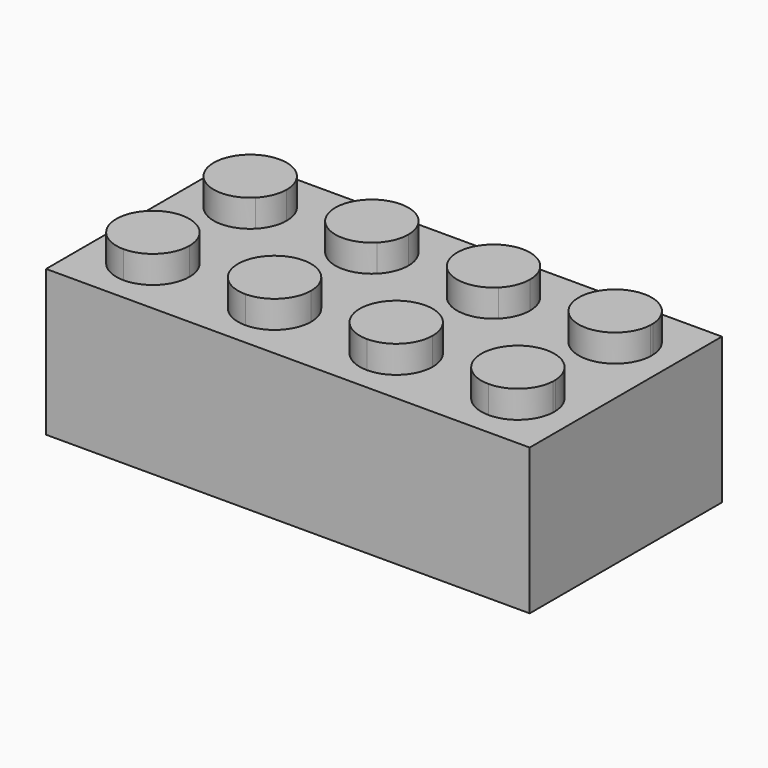
from build123d import *

# Parameters (mm, degrees)
F0_W     = 31.8
F0_H     = 15.8
F1_DEPTH = 9.6
F0_R     = 2.4
F0_W_2   = 0.3
F0_H_2   = 0.6
F2_DEPTH = 1
F3_DEPTH = 1.8
F4_DEPTH = 9.6


# Not quite as in the source:
# - a feature of the source that left no trace in its solid (it failed there, or was rolled back) is left out


with BuildPart() as f1:
    # F0 (on Top) → F1 (new body)
    with BuildSketch(Plane.XY):
        Rectangle(F0_W, F0_H)
        Polygon((-11.6973772652, 6.7), (-4.2973772652, 6.7), (-3.6973772652, 6.7), (3.7026227348, 6.7), (4.3026227348, 6.7), (11.7026227348, 6.7), (12.3026227348, 6.7), (14.7, 6.7), (14.7, 4.3), (14.7, 3.7), (14.7, -3.7), (14.7, -4.3), (14.7, -6.7), (12.3026227348, -6.7), (11.7026227348, -6.7), (4.3026227348, -6.7), (3.7026227348, -6.7), (-3.6973772652, -6.7), (-4.2973772652, -6.7), (-11.6973772652, -6.7), (-12.2973772652, -6.7), (-14.7, -6.7), (-14.7, -4.3), (-14.7, -3.7), (-14.7, 3.7), (-14.7, 4.3), (-14.7, 6.7), (-12.2973772652, 6.7), align=None, mode=Mode.SUBTRACT)
    extrude(amount=-F1_DEPTH)

    # F0 (on Top) → F2 (join)
    with BuildSketch(Plane.XY):
        with BuildLine():
            ThreePointArc((-2.3008776231, -2.3023872749), (1.2461276694, -3.0070235835), (3.255, 0))
            ThreePointArc((3.255, 0), (1.2461276864, 3.0070235764), (-2.3008775971, 2.3023873009))
            ThreePointArc((-2.3008775971, 2.3023873009), (-3.255, 1.84e-08), (-2.3008776231, -2.3023872749))
        make_face()
        Circle(F0_R, mode=Mode.SUBTRACT)
        with BuildLine():
            ThreePointArc((-2.3008775971, 2.3023873009), (1.2461276864, 3.0070235764), (3.255, 0))
            ThreePointArc((3.255, 0), (1.2461276694, -3.0070235835), (-2.3008776231, -2.3023872749))
            ThreePointArc((-2.3008776231, -2.3023872749), (-1.780217016, -3.0811961964), (-1.5973772652, -4))
            ThreePointArc((-1.5973772652, -4), (-2.3003209903, -5.6970562748), (-3.9973772652, -6.4))
            Line((-3.9973772652, -6.4), (-3.6973772652, -6.4))
            Line((-3.6973772652, -6.4), (-3.6973772652, -6.7))
            Line((-3.6973772652, -6.7), (3.7026227348, -6.7))
            Line((3.7026227348, -6.7), (3.7026227348, -6.4))
            Line((3.7026227348, -6.4), (4.0026227348, -6.4))
            ThreePointArc((4.0026227348, -6.4), (1.7851612895, -3.0819233484), (5.6991223839, -2.3023872819))
            ThreePointArc((5.6991223839, -2.3023872819), (4.745, 5e-09), (5.699122391, 2.3023872889))
            ThreePointArc((5.699122391, 2.3023872889), (1.7851612914, 3.0819233438), (4.0026227348, 6.4))
            Line((4.0026227348, 6.4), (3.7026227348, 6.4))
            Line((3.7026227348, 6.4), (3.7026227348, 6.7))
            Line((3.7026227348, 6.7), (-3.6973772652, 6.7))
            Line((-3.6973772652, 6.7), (-3.6973772652, 6.4))
            Line((-3.6973772652, 6.4), (-3.9973772652, 6.4))
            ThreePointArc((-3.9973772652, 6.4), (-2.3003209903, 5.6970562748), (-1.5973772652, 4))
            ThreePointArc((-1.5973772652, 4), (-1.7802170089, 3.0811962134), (-2.3008775971, 2.3023873009))
        make_face()
        with BuildLine():
            ThreePointArc((-2.3008776231, -2.3023872749), (-3.255, 1.84e-08), (-2.3008775971, 2.3023873009))
            ThreePointArc((-2.3008775971, 2.3023873009), (-6.2148387054, 3.0819233359), (-3.9973772652, 6.4))
            Line((-3.9973772652, 6.4), (-4.2973772652, 6.4))
            Line((-4.2973772652, 6.4), (-4.2973772652, 6.7))
            Line((-4.2973772652, 6.7), (-11.6973772652, 6.7))
            Line((-11.6973772652, 6.7), (-11.6973772652, 6.4))
            Line((-11.6973772652, 6.4), (-11.9973772652, 6.4))
            ThreePointArc((-11.9973772652, 6.4), (-10.3003209903, 5.6970562748), (-9.5973772652, 4))
            ThreePointArc((-9.5973772652, 4), (-9.780217011, 3.0811962084), (-10.3008776047, 2.3023872933))
            ThreePointArc((-10.3008776047, 2.3023872933), (-6.7538723186, 3.0070235785), (-4.745, 0))
            ThreePointArc((-4.745, 0), (-6.7538723174, -3.007023578), (-10.3008776029, -2.3023872951))
            ThreePointArc((-10.3008776029, -2.3023872951), (-9.7802170105, -3.0811962096), (-9.5973772652, -4))
            ThreePointArc((-9.5973772652, -4), (-10.3003209903, -5.6970562748), (-11.9973772652, -6.4))
            Line((-11.9973772652, -6.4), (-11.6973772652, -6.4))
            Line((-11.6973772652, -6.4), (-11.6973772652, -6.7))
            Line((-11.6973772652, -6.7), (-4.2973772652, -6.7))
            Line((-4.2973772652, -6.7), (-4.2973772652, -6.4))
            Line((-4.2973772652, -6.4), (-3.9973772652, -6.4))
            ThreePointArc((-3.9973772652, -6.4), (-6.2148387124, -3.0819233529), (-2.3008776231, -2.3023872749))
        make_face()
        with BuildLine():
            ThreePointArc((-3.9973772652, 6.4), (-6.2148387054, 3.0819233359), (-2.3008775971, 2.3023873009))
            ThreePointArc((-2.3008775971, 2.3023873009), (-1.7802170089, 3.0811962134), (-1.5973772652, 4))
            ThreePointArc((-1.5973772652, 4), (-2.3003209903, 5.6970562748), (-3.9973772652, 6.4))
        make_face()
        with BuildLine():
            ThreePointArc((-1.5973772652, -4), (-1.780217016, -3.0811961964), (-2.3008776231, -2.3023872749))
            ThreePointArc((-2.3008776231, -2.3023872749), (-6.2148387124, -3.0819233529), (-3.9973772652, -6.4))
            ThreePointArc((-3.9973772652, -6.4), (-2.3003209903, -5.6970562748), (-1.5973772652, -4))
        make_face()
        Polygon((-4.2973772652, 6.4), (-3.9973772652, 6.4), (-3.6973772652, 6.4), (-3.6973772652, 6.7), (-4.2973772652, 6.7), align=None)
        Polygon((-3.6973772652, -6.4), (-3.9973772652, -6.4), (-4.2973772652, -6.4), (-4.2973772652, -6.7), (-3.6973772652, -6.7), align=None)
        Polygon((-11.6973772652, 6.4), (-11.6973772652, 6.7), (-12.2973772652, 6.7), (-12.2973772652, 6.4), (-11.9973772652, 6.4), align=None)
        Polygon((4.3026227348, 6.7), (3.7026227348, 6.7), (3.7026227348, 6.4), (4.0026227348, 6.4), (4.3026227348, 6.4), align=None)
        Polygon((-12.2973772652, -6.7), (-11.6973772652, -6.7), (-11.6973772652, -6.4), (-11.9973772652, -6.4), (-12.2973772652, -6.4), align=None)
        Polygon((3.7026227348, -6.4), (3.7026227348, -6.7), (4.3026227348, -6.7), (4.3026227348, -6.4), (4.0026227348, -6.4), align=None)
        with BuildLine():
            Line((-12.2973772652, 6.4), (-12.2973772652, 6.7))
            Line((-12.2973772652, 6.7), (-14.7, 6.7))
            Line((-14.7, 6.7), (-14.7, 4.3))
            Line((-14.7, 4.3), (-14.4, 4.3))
            Line((-14.4, 4.3), (-14.4, 3.7))
            Line((-14.4, 3.7), (-14.7, 3.7))
            Line((-14.7, 3.7), (-14.7, -3.7))
            Line((-14.7, -3.7), (-14.4, -3.7))
            Line((-14.4, -3.7), (-14.4, -4.3))
            Line((-14.4, -4.3), (-14.7, -4.3))
            Line((-14.7, -4.3), (-14.7, -6.7))
            Line((-14.7, -6.7), (-12.2973772652, -6.7))
            Line((-12.2973772652, -6.7), (-12.2973772652, -6.4))
            Line((-12.2973772652, -6.4), (-11.9973772652, -6.4))
            ThreePointArc((-11.9973772652, -6.4), (-14.214838707, -3.0819233398), (-10.3008776029, -2.3023872951))
            ThreePointArc((-10.3008776029, -2.3023872951), (-11.255, -1.3e-09), (-10.3008776047, 2.3023872933))
            ThreePointArc((-10.3008776047, 2.3023872933), (-14.2148387075, 3.0819233409), (-11.9973772652, 6.4))
            Line((-11.9973772652, 6.4), (-12.2973772652, 6.4))
        make_face()
        with BuildLine():
            Line((11.7026227348, 6.7), (4.3026227348, 6.7))
            Line((4.3026227348, 6.7), (4.3026227348, 6.4))
            Line((4.3026227348, 6.4), (4.0026227348, 6.4))
            ThreePointArc((4.0026227348, 6.4), (5.6996790097, 5.6970562748), (6.4026227348, 4))
            ThreePointArc((6.4026227348, 4), (6.2197829878, 3.0811962056), (5.699122391, 2.3023872889))
            ThreePointArc((5.699122391, 2.3023872889), (9.2461276786, 3.0070235797), (11.255, 0))
            ThreePointArc((11.255, 0), (9.246127674, -3.0070235816), (5.6991223839, -2.3023872819))
            ThreePointArc((5.6991223839, -2.3023872819), (6.2197829859, -3.081196201), (6.4026227348, -4))
            ThreePointArc((6.4026227348, -4), (5.6996790097, -5.6970562748), (4.0026227348, -6.4))
            Line((4.0026227348, -6.4), (4.3026227348, -6.4))
            Line((4.3026227348, -6.4), (4.3026227348, -6.7))
            Line((4.3026227348, -6.7), (11.7026227348, -6.7))
            Line((11.7026227348, -6.7), (11.7026227348, -6.4))
            Line((11.7026227348, -6.4), (12.0026227348, -6.4))
            ThreePointArc((12.0026227348, -6.4), (10.2663610188, -2.3430765699), (14.4, -3.8878293777))
            Line((14.4, -3.8878293777), (14.4, -3.7))
            Line((14.4, -3.7), (14.7, -3.7))
            Line((14.7, -3.7), (14.7, 3.7))
            Line((14.7, 3.7), (14.4, 3.7))
            Line((14.4, 3.7), (14.4, 3.8878293777))
            ThreePointArc((14.4, 3.8878293777), (10.2663610188, 2.3430765699), (12.0026227348, 6.4))
            Line((12.0026227348, 6.4), (11.7026227348, 6.4))
            Line((11.7026227348, 6.4), (11.7026227348, 6.7))
        make_face()
        with BuildLine():
            ThreePointArc((-9.5973772652, 4), (-10.3003209903, 5.6970562748), (-11.9973772652, 6.4))
            ThreePointArc((-11.9973772652, 6.4), (-14.2148387075, 3.0819233409), (-10.3008776047, 2.3023872933))
            ThreePointArc((-10.3008776047, 2.3023872933), (-9.780217011, 3.0811962084), (-9.5973772652, 4))
        make_face()
        Polygon((12.3026227348, 6.7), (11.7026227348, 6.7), (11.7026227348, 6.4), (12.0026227348, 6.4), (12.3026227348, 6.4), align=None)
        with BuildLine():
            ThreePointArc((6.4026227348, 4), (5.6996790097, 5.6970562748), (4.0026227348, 6.4))
            ThreePointArc((4.0026227348, 6.4), (1.7851612914, 3.0819233438), (5.699122391, 2.3023872889))
            ThreePointArc((5.699122391, 2.3023872889), (6.2197829878, 3.0811962056), (6.4026227348, 4))
        make_face()
        with BuildLine():
            ThreePointArc((-10.3008776029, -2.3023872951), (-14.214838707, -3.0819233398), (-11.9973772652, -6.4))
            ThreePointArc((-11.9973772652, -6.4), (-10.3003209903, -5.6970562748), (-9.5973772652, -4))
            ThreePointArc((-9.5973772652, -4), (-9.7802170105, -3.0811962096), (-10.3008776029, -2.3023872951))
        make_face()
        Polygon((11.7026227348, -6.4), (11.7026227348, -6.7), (12.3026227348, -6.7), (12.3026227348, -6.4), (12.0026227348, -6.4), align=None)
        with BuildLine():
            ThreePointArc((5.6991223839, -2.3023872819), (1.7851612895, -3.0819233484), (4.0026227348, -6.4))
            ThreePointArc((4.0026227348, -6.4), (5.6996790097, -5.6970562748), (6.4026227348, -4))
            ThreePointArc((6.4026227348, -4), (6.2197829859, -3.081196201), (5.6991223839, -2.3023872819))
        make_face()
        with Locations((-14.55, 4)):
            Rectangle(F0_W_2, F0_H_2)
        with BuildLine():
            ThreePointArc((-4.745, 0), (-6.7538723186, 3.0070235785), (-10.3008776047, 2.3023872933))
            ThreePointArc((-10.3008776047, 2.3023872933), (-11.255, -1.3e-09), (-10.3008776029, -2.3023872951))
            ThreePointArc((-10.3008776029, -2.3023872951), (-6.7538723174, -3.007023578), (-4.745, 0))
        make_face()
        with Locations((-8, 0)):
            Circle(F0_R, mode=Mode.SUBTRACT)
        with BuildLine():
            Line((14.7, 6.7), (12.3026227348, 6.7))
            Line((12.3026227348, 6.7), (12.3026227348, 6.4))
            Line((12.3026227348, 6.4), (12.0026227348, 6.4))
            ThreePointArc((12.0026227348, 6.4), (13.659546165, 5.7362617161), (14.4, 4.1121706223))
            Line((14.4, 4.1121706223), (14.4, 4.3))
            Line((14.4, 4.3), (14.7, 4.3))
            Line((14.7, 4.3), (14.7, 6.7))
        make_face()
        with BuildLine():
            ThreePointArc((11.255, 0), (9.2461276786, 3.0070235797), (5.699122391, 2.3023872889))
            ThreePointArc((5.699122391, 2.3023872889), (4.745, 5e-09), (5.6991223839, -2.3023872819))
            ThreePointArc((5.6991223839, -2.3023872819), (9.246127674, -3.0070235816), (11.255, 0))
        make_face()
        with Locations((8, 0)):
            Circle(F0_R, mode=Mode.SUBTRACT)
        with Locations((-14.55, -4)):
            Rectangle(F0_W_2, F0_H_2)
        with BuildLine():
            Line((12.3026227348, -6.4), (12.3026227348, -6.7))
            Line((12.3026227348, -6.7), (14.7, -6.7))
            Line((14.7, -6.7), (14.7, -4.3))
            Line((14.7, -4.3), (14.4, -4.3))
            Line((14.4, -4.3), (14.4, -4.1121706223))
            ThreePointArc((14.4, -4.1121706223), (13.659546165, -5.7362617161), (12.0026227348, -6.4))
            Line((12.0026227348, -6.4), (12.3026227348, -6.4))
        make_face()
        with BuildLine():
            ThreePointArc((14.4, 4.1121706223), (13.659546165, 5.7362617161), (12.0026227348, 6.4))
            ThreePointArc((12.0026227348, 6.4), (10.2663610188, 2.3430765699), (14.4, 3.8878293777))
            Line((14.4, 3.8878293777), (14.4, 4.1121706223))
        make_face()
        with BuildLine():
            ThreePointArc((14.4, -3.8878293777), (10.2663610188, -2.3430765699), (12.0026227348, -6.4))
            ThreePointArc((12.0026227348, -6.4), (13.659546165, -5.7362617161), (14.4, -4.1121706223))
            Line((14.4, -4.1121706223), (14.4, -3.8878293777))
        make_face()
        with BuildLine():
            Line((14.7, 3.7), (14.7, 4.3))
            Line((14.7, 4.3), (14.4, 4.3))
            Line((14.4, 4.3), (14.4, 4.1121706223))
            ThreePointArc((14.4, 4.1121706223), (14.4019669615, 4.05610064), (14.4026227348, 4))
            ThreePointArc((14.4026227348, 4), (14.4019669615, 3.94389936), (14.4, 3.8878293777))
            Line((14.4, 3.8878293777), (14.4, 3.7))
            Line((14.4, 3.7), (14.7, 3.7))
        make_face()
        with BuildLine():
            Line((14.4, -4.3), (14.7, -4.3))
            Line((14.7, -4.3), (14.7, -3.7))
            Line((14.7, -3.7), (14.4, -3.7))
            Line((14.4, -3.7), (14.4, -3.8878293777))
            ThreePointArc((14.4, -3.8878293777), (14.4019669615, -3.94389936), (14.4026227348, -4))
            ThreePointArc((14.4026227348, -4), (14.4019669615, -4.05610064), (14.4, -4.1121706223))
            Line((14.4, -4.1121706223), (14.4, -4.3))
        make_face()
        Circle(F0_R)
        with Locations((8, 0)):
            Circle(F0_R)
        with Locations((-8, 0)):
            Circle(F0_R)
    extrude(amount=-F2_DEPTH)

    # F0 (on Top) → F3 (join)
    with BuildSketch(Plane.XY):
        with BuildLine():
            ThreePointArc((-3.9973772652, 6.4), (-6.2148387054, 3.0819233359), (-2.3008775971, 2.3023873009))
            ThreePointArc((-2.3008775971, 2.3023873009), (-1.7802170089, 3.0811962134), (-1.5973772652, 4))
            ThreePointArc((-1.5973772652, 4), (-2.3003209903, 5.6970562748), (-3.9973772652, 6.4))
        make_face()
        with BuildLine():
            ThreePointArc((-1.5973772652, -4), (-1.780217016, -3.0811961964), (-2.3008776231, -2.3023872749))
            ThreePointArc((-2.3008776231, -2.3023872749), (-6.2148387124, -3.0819233529), (-3.9973772652, -6.4))
            ThreePointArc((-3.9973772652, -6.4), (-2.3003209903, -5.6970562748), (-1.5973772652, -4))
        make_face()
        with BuildLine():
            ThreePointArc((-9.5973772652, 4), (-10.3003209903, 5.6970562748), (-11.9973772652, 6.4))
            ThreePointArc((-11.9973772652, 6.4), (-14.2148387075, 3.0819233409), (-10.3008776047, 2.3023872933))
            ThreePointArc((-10.3008776047, 2.3023872933), (-9.780217011, 3.0811962084), (-9.5973772652, 4))
        make_face()
        with BuildLine():
            ThreePointArc((6.4026227348, 4), (5.6996790097, 5.6970562748), (4.0026227348, 6.4))
            ThreePointArc((4.0026227348, 6.4), (1.7851612914, 3.0819233438), (5.699122391, 2.3023872889))
            ThreePointArc((5.699122391, 2.3023872889), (6.2197829878, 3.0811962056), (6.4026227348, 4))
        make_face()
        with BuildLine():
            ThreePointArc((-10.3008776029, -2.3023872951), (-14.214838707, -3.0819233398), (-11.9973772652, -6.4))
            ThreePointArc((-11.9973772652, -6.4), (-10.3003209903, -5.6970562748), (-9.5973772652, -4))
            ThreePointArc((-9.5973772652, -4), (-9.7802170105, -3.0811962096), (-10.3008776029, -2.3023872951))
        make_face()
        with BuildLine():
            ThreePointArc((5.6991223839, -2.3023872819), (1.7851612895, -3.0819233484), (4.0026227348, -6.4))
            ThreePointArc((4.0026227348, -6.4), (5.6996790097, -5.6970562748), (6.4026227348, -4))
            ThreePointArc((6.4026227348, -4), (6.2197829859, -3.081196201), (5.6991223839, -2.3023872819))
        make_face()
        with BuildLine():
            ThreePointArc((14.4, 4.1121706223), (13.659546165, 5.7362617161), (12.0026227348, 6.4))
            ThreePointArc((12.0026227348, 6.4), (10.2663610188, 2.3430765699), (14.4, 3.8878293777))
            Line((14.4, 3.8878293777), (14.4, 4.1121706223))
        make_face()
        with BuildLine():
            ThreePointArc((14.4, -3.8878293777), (10.2663610188, -2.3430765699), (12.0026227348, -6.4))
            ThreePointArc((12.0026227348, -6.4), (13.659546165, -5.7362617161), (14.4, -4.1121706223))
            Line((14.4, -4.1121706223), (14.4, -3.8878293777))
        make_face()
    extrude(amount=F3_DEPTH)

    # F0 (on Top) → F4 (join)
    with BuildSketch(Plane.XY):
        Polygon((11.7026227348, -6.4), (11.7026227348, -6.7), (12.3026227348, -6.7), (12.3026227348, -6.4), (12.0026227348, -6.4), align=None)
        Polygon((12.3026227348, 6.7), (11.7026227348, 6.7), (11.7026227348, 6.4), (12.0026227348, 6.4), (12.3026227348, 6.4), align=None)
        Polygon((4.3026227348, 6.7), (3.7026227348, 6.7), (3.7026227348, 6.4), (4.0026227348, 6.4), (4.3026227348, 6.4), align=None)
        Polygon((-4.2973772652, 6.4), (-3.9973772652, 6.4), (-3.6973772652, 6.4), (-3.6973772652, 6.7), (-4.2973772652, 6.7), align=None)
        Polygon((-11.6973772652, 6.4), (-11.6973772652, 6.7), (-12.2973772652, 6.7), (-12.2973772652, 6.4), (-11.9973772652, 6.4), align=None)
        with Locations((-14.55, 4)):
            Rectangle(F0_W_2, F0_H_2)
        with Locations((-14.55, -4)):
            Rectangle(F0_W_2, F0_H_2)
        Polygon((-12.2973772652, -6.7), (-11.6973772652, -6.7), (-11.6973772652, -6.4), (-11.9973772652, -6.4), (-12.2973772652, -6.4), align=None)
        Polygon((-3.6973772652, -6.4), (-3.9973772652, -6.4), (-4.2973772652, -6.4), (-4.2973772652, -6.7), (-3.6973772652, -6.7), align=None)
        Polygon((3.7026227348, -6.4), (3.7026227348, -6.7), (4.3026227348, -6.7), (4.3026227348, -6.4), (4.0026227348, -6.4), align=None)
        with BuildLine():
            ThreePointArc((11.255, 0), (9.2461276786, 3.0070235797), (5.699122391, 2.3023872889))
            ThreePointArc((5.699122391, 2.3023872889), (4.745, 5e-09), (5.6991223839, -2.3023872819))
            ThreePointArc((5.6991223839, -2.3023872819), (9.246127674, -3.0070235816), (11.255, 0))
        make_face()
        with Locations((8, 0)):
            Circle(F0_R, mode=Mode.SUBTRACT)
        with BuildLine():
            ThreePointArc((-2.3008776231, -2.3023872749), (1.2461276694, -3.0070235835), (3.255, 0))
            ThreePointArc((3.255, 0), (1.2461276864, 3.0070235764), (-2.3008775971, 2.3023873009))
            ThreePointArc((-2.3008775971, 2.3023873009), (-3.255, 1.84e-08), (-2.3008776231, -2.3023872749))
        make_face()
        Circle(F0_R, mode=Mode.SUBTRACT)
        with BuildLine():
            ThreePointArc((-4.745, 0), (-6.7538723186, 3.0070235785), (-10.3008776047, 2.3023872933))
            ThreePointArc((-10.3008776047, 2.3023872933), (-11.255, -1.3e-09), (-10.3008776029, -2.3023872951))
            ThreePointArc((-10.3008776029, -2.3023872951), (-6.7538723174, -3.007023578), (-4.745, 0))
        make_face()
        with Locations((-8, 0)):
            Circle(F0_R, mode=Mode.SUBTRACT)
        with BuildLine():
            Line((14.4, -4.3), (14.7, -4.3))
            Line((14.7, -4.3), (14.7, -3.7))
            Line((14.7, -3.7), (14.4, -3.7))
            Line((14.4, -3.7), (14.4, -3.8878293777))
            ThreePointArc((14.4, -3.8878293777), (14.4019669615, -3.94389936), (14.4026227348, -4))
            ThreePointArc((14.4026227348, -4), (14.4019669615, -4.05610064), (14.4, -4.1121706223))
            Line((14.4, -4.1121706223), (14.4, -4.3))
        make_face()
    extrude(amount=-F4_DEPTH)


solid = f1.part
